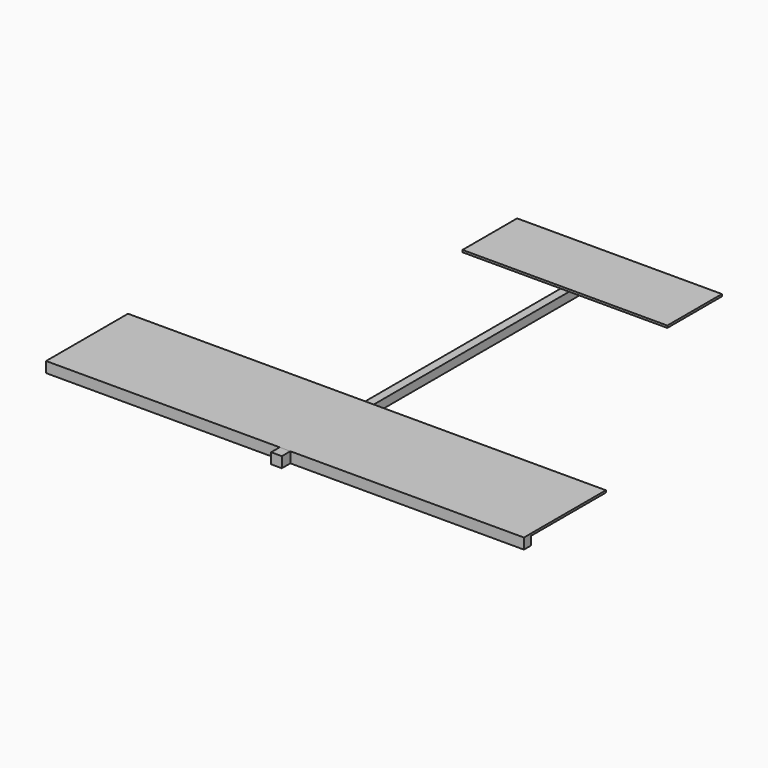
from build123d import *

# Parameters (mm, degrees)
F0_W      = 6.35
F0_H      = 6.35
F1_DEPTH  = 304.8
F2_W      = 73.025
F2_H      = 50.8
F2_W_2    = 6.35
F3_DEPTH  = 1.5875
F4_W      = 6.35
F4_H      = 69.85
F5_DEPTH  = 1.5875
F7_DEPTH  = 6.35
F9_DEPTH  = 6.35
F11_W     = 7.9375
F11_H     = 7.9375
F12_DEPTH = 7.9375


# Not quite as in the source:
# - a length typed as a fraction of an inch, garbled in the dataset ("3 / 203.2 mm" for 3/8 in), is restored


with BuildPart() as f1:
    # F0 (on Front) → F1 (new body)
    with BuildSketch(Plane.XZ):
        Rectangle(F0_W, F0_H)
    extrude(amount=F1_DEPTH)

    # F2 (on face) → F3 (join)
    with BuildSketch(Plane.XY.offset(3.175)):
        with Locations((39.6875, -25.4)):
            Rectangle(F2_W, F2_H)
        with Locations((-39.6875, -25.4)):
            Rectangle(F2_W, F2_H)
        with Locations((0, -25.4)):
            Rectangle(F2_W_2, F2_H)
    extrude(amount=F3_DEPTH)

    # F4 (on face) → F5 (join)
    with BuildSketch(Plane.XY.offset(3.175)):
        Polygon((-3.175, -234.95), (-177.8, -234.95), (-177.8, -311.15), (177.8, -311.15), (177.8, -234.95), (3.175, -234.95), (3.175, -304.8), (-3.175, -304.8), align=None)
        with Locations((0, -269.875)):
            Rectangle(F4_W, F4_H)
    extrude(amount=F5_DEPTH)

    # F6 (on face) → F7 (join)
    with BuildSketch(Plane(origin=(0, 0, 3.175), x_dir=(1, 0, 0), z_dir=(0, 0, -1))):
        Polygon((-177.8, 311.15), (-177.8, 304.8), (-3.175, 304.8), (3.175, 304.8), (177.8, 304.8), (177.8, 311.15), align=None)
    extrude(amount=F7_DEPTH)

    # F8 (on face) → F9 (join)
    with BuildSketch(Plane(origin=(0, 0, 3.175), x_dir=(1, 0, 0), z_dir=(0, 0, -1))):
        Polygon((-177.8, 304.8), (-3.175, 234.95), (-3.175, 241.7891593051), (-160.7021017373, 304.8), align=None)
    extrude(amount=F9_DEPTH)

    # F10: F1 across plane


with BuildPart() as f1_1:
    add(f1.part)
    add(f1.part.mirror(Plane.YZ))


with BuildPart() as f12:
    # F11 (on face) → F12 (new body)
    with BuildSketch(Plane.XZ.offset(311.15)):
        with Locations((0, 0.79375)):
            Rectangle(F11_W, F11_H)
    extrude(amount=F12_DEPTH)


solid = Compound([f1_1.part, f12.part])
